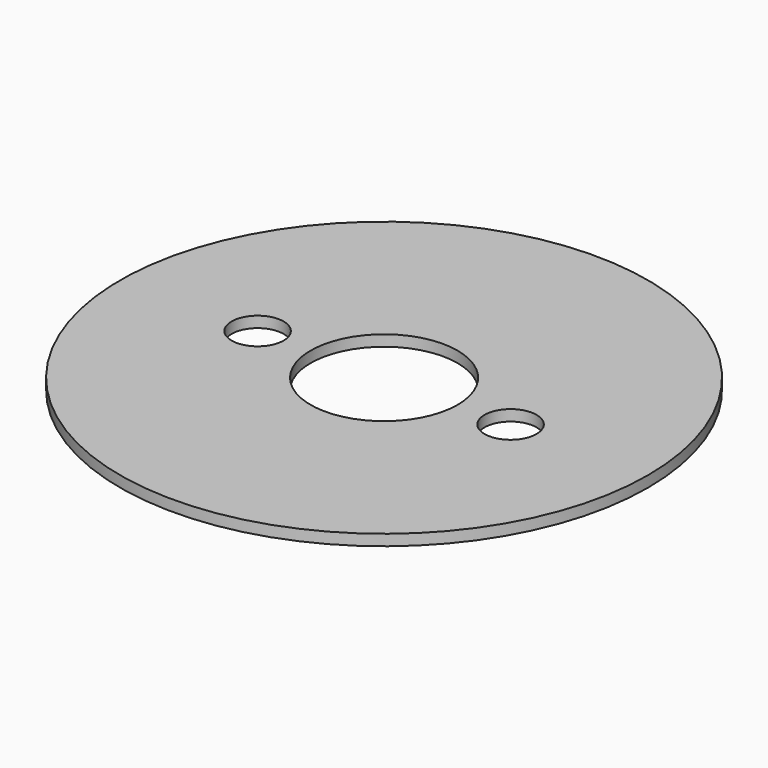
from build123d import *

# Parameters (mm, degrees)
F0_R     = 38.1
F0_R_2   = 3.75
F0_R_3   = 10.60685
F1_DEPTH = 1.5875


# Not quite as in the source:
# - a length typed as a fraction of an inch, garbled in the dataset ("3 / 203.2 mm" for 3/8 in), is restored


with BuildPart() as f1:
    # F0 (on Top) → F1 (new body)
    with BuildSketch(Plane.XY):
        Circle(F0_R)
        with Locations((-18.25625, 0)):
            Circle(F0_R_2, mode=Mode.SUBTRACT)
        Circle(F0_R_3, mode=Mode.SUBTRACT)
        with Locations((18.25625, 0)):
            Circle(F0_R_2, mode=Mode.SUBTRACT)
    extrude(amount=F1_DEPTH)


solid = f1.part
